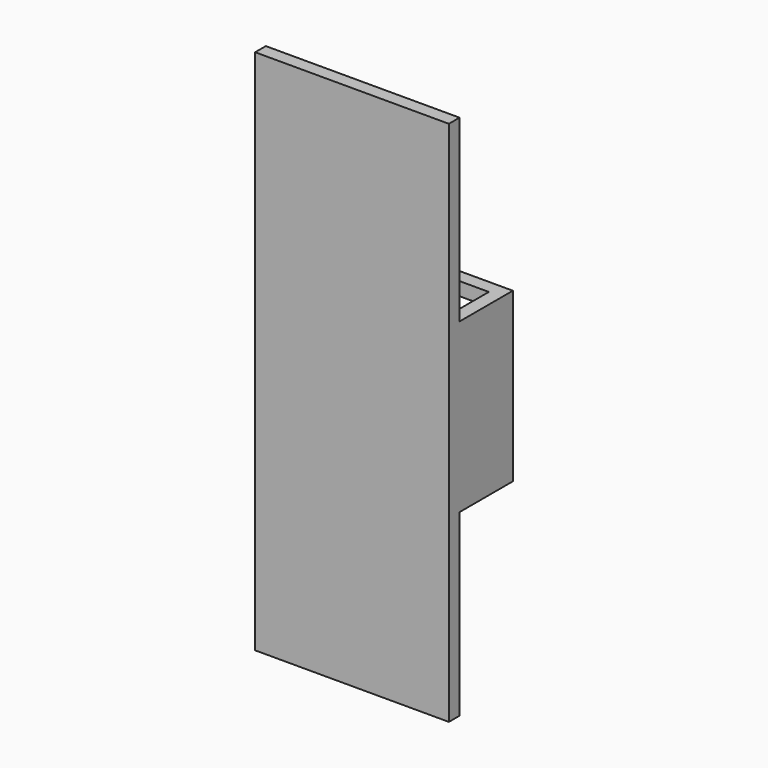
from build123d import *

# Parameters (mm, degrees)
F0_W     = 36.92906
F0_H     = 100.3808
F1_DEPTH = 2.54
F2_W     = 36.92906
F2_H     = 31.99892
F3_DEPTH = 15.24
F4_T     = -2.54
F5_W     = 31.84906
F5_H     = 26.91892
F6_DEPTH = 2.54


# Not quite as in the source:
# - a shell that OpenCascade refuses in one call is made with other operations: the cavity is built on its own and cut out


with BuildPart() as f1:
    # F0 (on Front) → F1 (new body)
    with BuildSketch(Plane.XZ):
        with Locations((-3.5625953953, 0.4117265198)):
            Rectangle(F0_W, F0_H)
    extrude(amount=F1_DEPTH)

    # F2 (on face) → F3 (join)
    with BuildSketch(Plane.XZ.offset(2.54)):
        with Locations((-3.5625953953, 0.3964865198)):
            Rectangle(F2_W, F2_H)
    extrude(amount=-F3_DEPTH)

    # F4: a shell. OpenCascade refuses it in one call, so the cavity is built on its own and cut out:
    # the body offset inwards by the wall thickness, plus a prism from it out through each open face.
    f4_core = offset(f1.part, amount=F4_T, kind=Kind.INTERSECTION, mode=Mode.PRIVATE)
    f4_exits = [f4_core.faces().sort_by_distance(p)[0] for p in [
        (-3.562595, 5.08, 13.855947),
    ]]
    add(f4_core, mode=Mode.SUBTRACT)
    extrude(f4_exits, amount=-F4_T, mode=Mode.SUBTRACT)

    # F5 (on face) → F6 (cut, through all)
    with BuildSketch(Plane(origin=(0, 12.7, 0), x_dir=(-1, 0, 0), z_dir=(0, 1, 0))):
        with Locations((3.5625953953, 0.3964865198)):
            Rectangle(F5_W, F5_H)
    extrude(amount=-F6_DEPTH, mode=Mode.SUBTRACT)


solid = f1.part
